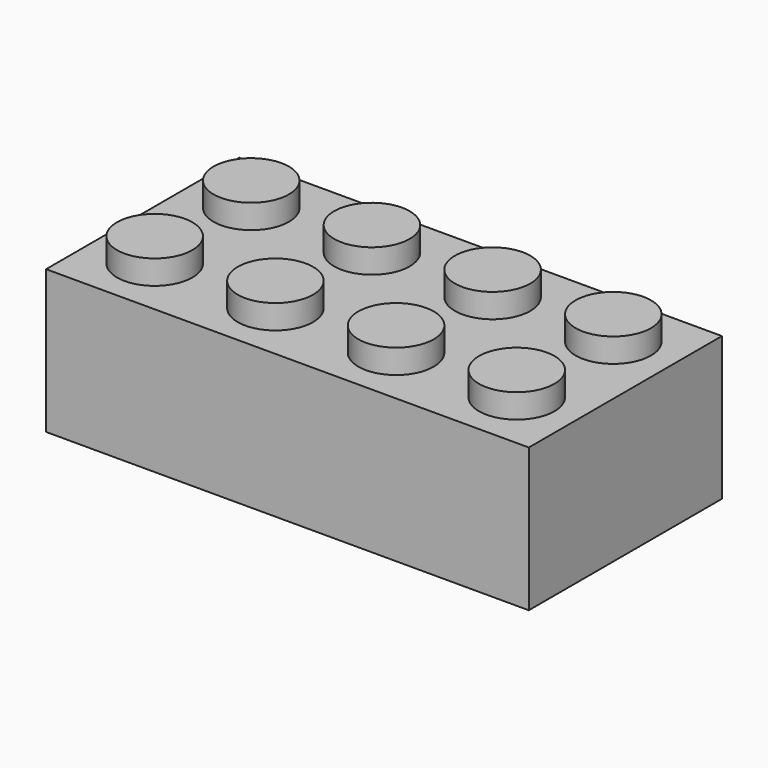
from build123d import *

# Parameters (mm, degrees)
F0_W          = 32
F0_H          = 16
F1_DEPTH      = 9.5
F2_R          = 2.5
F3_DEPTH      = 1.6
F5_T          = -1.5
F4_R          = 3.1568542495
F6_DEPTH      = 9.5
F7_T          = 1
F7_T3_DEPTH   = 10
F7_T5_DEPTH   = 15
F7_T7_DEPTH   = 31
F8_W          = 0.5
F8_H          = 4.8829936233
F9_DEPTH      = 9.5
F10_TEXT_SIZE = 4.2820941114
F11_DEPTH     = 0.7


# Not quite as in the source:
# - a shell that OpenCascade refuses in one call is made with other operations: the cavity is built on its own and cut out
# - Text() gives the source's letters only with a copy of the font that has no kerning and outlines rounded to 1/6400 em; it was checked with that copy


with BuildPart() as f1:
    # F0 (on Top) → F1 (new body)
    with BuildSketch(Plane.XY):
        Rectangle(F0_W, F0_H)
    extrude(amount=F1_DEPTH)

    # F2 (on face) → F3 (join)
    with BuildSketch(Plane.XY.offset(9.5)):
        with Locations((-12, 4)):
            Circle(F2_R)
        with Locations((-12, -4)):
            Circle(F2_R)
        with Locations((-4, 4)):
            Circle(F2_R)
        with Locations((-4, -4)):
            Circle(F2_R)
        with Locations((4, 4)):
            Circle(F2_R)
        with Locations((12, 4)):
            Circle(F2_R)
        with Locations((12, -4)):
            Circle(F2_R)
        with Locations((4, -4)):
            Circle(F2_R)
    extrude(amount=F3_DEPTH)

    # F5
    f5_openings = [f1.faces().sort_by_distance(p)[0] for p in [
        (0, 0, 0),
    ]]
    offset(amount=F5_T, openings=f5_openings, kind=Kind.INTERSECTION)

    # F4 (on face) → F6 (join)
    with BuildSketch(Plane.XY.offset(9.5)):
        Circle(F4_R)
        with Locations((-8, 0)):
            Circle(F4_R)
        with Locations((8, 0)):
            Circle(F4_R)
    extrude(amount=-F6_DEPTH)

    # F7: shell of thickness 1, made by hand


with BuildPart() as f7_core1:
    # F7_t2: copy of F1
    add(f1.part)

    # the walls: a layer under each face that stays
    f7_faces = [f7_core1.faces().sort_by_distance(p)[0] for p in [
        (0, 8, 4.75),
        (0, 0, 9.5),
        (9.5, 4, 10.3),
        (12, 4, 11.1),
        (-6.5, 4, 10.3),
        (-4, 4, 11.1),
        (1.5, 4, 10.3),
        (4, 4, 11.1),
        (1.5, -4, 10.3),
        (4, -4, 11.1),
        (-6.5, -4, 10.3),
        (-4, -4, 11.1),
        (-14.5, 4, 10.3),
        (-12, 4, 11.1),
        (9.5, -4, 10.3),
        (12, -4, 11.1),
        (-14.5, -4, 10.3),
        (-12, -4, 11.1),
        (0, -8, 4.75),
        (-13.7142857143, -6.8571428571, 0),
        (-14.5, 0, 4),
        (-9.6666666667, -4.3333333333, 8),
        (11, 4, 8.8),
        (12, 4, 9.6),
        (3, 4, 8.8),
        (4, 4, 9.6),
        (4.8431457505, 0, 4),
        (-3.1568542495, 0, 4),
        (-5, 4, 8.8),
        (-4, 4, 9.6),
        (-13, 4, 8.8),
        (-12, 4, 9.6),
        (-11.1568542495, 0, 4),
        (11, -4, 8.8),
        (12, -4, 9.6),
        (3, -4, 8.8),
        (4, -4, 9.6),
        (-5, -4, 8.8),
        (-4, -4, 9.6),
        (-13, -4, 8.8),
        (-12, -4, 9.6),
        (0, -6.5, 4),
        (14.5, 0, 4),
        (0, 6.5, 4),
        (-16, 0, 4.75),
        (16, 0, 4.75),
    ]]
    thicken(f7_faces, amount=-F7_T, mode=Mode.SUBTRACT)

    # F7_s4 → F7_t3 (cut)
    with BuildSketch(Plane.XY.offset(-1)):
        Polygon((-14.49, -6.49), (-15.5, -6.5), (-15.5, -7.5), (-14.5, -7.5), align=None)
        Polygon((-14.49, 6.49), (-15.5, 6.5), (-15.5, 7.5), (-14.5, 7.5), align=None)
        Polygon((14.49, -6.49), (14.5, -7.5), (15.5, -7.5), (15.5, -6.5), align=None)
        Polygon((14.49, 6.49), (15.5, 6.5), (15.5, 7.5), (14.5, 7.5), align=None)
    extrude(amount=F7_T3_DEPTH, mode=Mode.SUBTRACT)

    # F7_s6 → F7_t5 (cut)
    with BuildSketch(Plane.XZ.offset(-7.5)):
        Polygon((-14.49, 7.99), (-15.5, 8), (-15.5, 9), (-14.5, 9), align=None)
        Polygon((14.49, 7.99), (14.5, 9), (15.5, 9), (15.5, 8), align=None)
    extrude(amount=F7_T5_DEPTH, mode=Mode.SUBTRACT)

    # F7_s8 → F7_t7 (cut)
    with BuildSketch(Plane.YZ.offset(-15.5)):
        Polygon((-6.49, 7.99), (-6.5, 9), (-7.5, 9), (-7.5, 8), align=None)
        Polygon((6.49, 7.99), (6.5, 9), (7.5, 9), (7.5, 8), align=None)
    extrude(amount=F7_T7_DEPTH, mode=Mode.SUBTRACT)

    # F7_s9 → F7_t10 (revolve, cut)
    with BuildSketch(Plane.XZ.offset(4)):
        Polygon((-9.49, 9.51), (-9.5, 8.5), (-10.5, 8.5), (-10.5, 9.5), align=None)
    revolve(axis=Axis((-12, -4, 9.5), (0, 0, -1)), mode=Mode.SUBTRACT)

    # F7_s11 → F7_t12 (revolve, cut)
    with BuildSketch(Plane.XZ.offset(4)):
        Polygon((14.51, 9.51), (14.5, 8.5), (13.5, 8.5), (13.5, 9.5), align=None)
    revolve(axis=Axis((12, -4, 9.5), (0, 0, -1)), mode=Mode.SUBTRACT)

    # F7_s13 → F7_t14 (revolve, cut)
    with BuildSketch(Plane.XZ.offset(-4)):
        Polygon((-9.49, 9.51), (-9.5, 8.5), (-10.5, 8.5), (-10.5, 9.5), align=None)
    revolve(axis=Axis((-12, 4, 9.5), (0, 0, -1)), mode=Mode.SUBTRACT)

    # F7_s15 → F7_t16 (revolve, cut)
    with BuildSketch(Plane.XZ.offset(4)):
        Polygon((-1.49, 9.51), (-1.5, 8.5), (-2.5, 8.5), (-2.5, 9.5), align=None)
    revolve(axis=Axis((-4, -4, 9.5), (0, 0, -1)), mode=Mode.SUBTRACT)

    # F7_s17 → F7_t18 (revolve, cut)
    with BuildSketch(Plane.XZ.offset(4)):
        Polygon((6.51, 9.51), (6.5, 8.5), (5.5, 8.5), (5.5, 9.5), align=None)
    revolve(axis=Axis((4, -4, 9.5), (0, 0, -1)), mode=Mode.SUBTRACT)

    # F7_s19 → F7_t20 (revolve, cut)
    with BuildSketch(Plane.XZ.offset(-4)):
        Polygon((6.51, 9.51), (6.5, 8.5), (5.5, 8.5), (5.5, 9.5), align=None)
    revolve(axis=Axis((4, 4, 9.5), (0, 0, -1)), mode=Mode.SUBTRACT)

    # F7_s21 → F7_t22 (revolve, cut)
    with BuildSketch(Plane.XZ.offset(-4)):
        Polygon((-1.49, 9.51), (-1.5, 8.5), (-2.5, 8.5), (-2.5, 9.5), align=None)
    revolve(axis=Axis((-4, 4, 9.5), (0, 0, -1)), mode=Mode.SUBTRACT)

    # F7_s23 → F7_t24 (revolve, cut)
    with BuildSketch(Plane.XZ.offset(-4)):
        Polygon((14.51, 9.51), (14.5, 8.5), (13.5, 8.5), (13.5, 9.5), align=None)
    revolve(axis=Axis((12, 4, 9.5), (0, 0, -1)), mode=Mode.SUBTRACT)

    # F7_s25 → F7_t26 (revolve, cut)
    with BuildSketch(Plane.XZ):
        Polygon((-4.8331457505, 7.99), (-4.8431457505, 9), (-5.8431457505, 9), (-5.8431457505, 8), align=None)
    revolve(axis=Axis((-8, 0, 8), (0, 0, 1)), mode=Mode.SUBTRACT)

    # F7_s27 → F7_t28 (revolve, cut)
    with BuildSketch(Plane.XZ):
        Polygon((3.1668542495, 7.99), (3.1568542495, 9), (2.1568542495, 9), (2.1568542495, 8), align=None)
    revolve(axis=Axis((0, 0, 8), (0, 0, 1)), mode=Mode.SUBTRACT)

    # F7_s29 → F7_t30 (revolve, cut)
    with BuildSketch(Plane.XZ):
        Polygon((11.1668542495, 7.99), (11.1568542495, 9), (10.1568542495, 9), (10.1568542495, 8), align=None)
    revolve(axis=Axis((8, 0, 8), (0, 0, 1)), mode=Mode.SUBTRACT)

    # F7_s31 → F7_t32 (revolve, cut)
    with BuildSketch(Plane.XZ.offset(-4)):
        Polygon((12.99, 9.59), (14, 9.6), (14, 10.6), (13, 10.6), align=None)
    revolve(axis=Axis((12, 4, 9.6), (0, 0, -1)), mode=Mode.SUBTRACT)

    # F7_s33 → F7_t34 (revolve, cut)
    with BuildSketch(Plane.XZ.offset(-4)):
        Polygon((4.99, 9.59), (6, 9.6), (6, 10.6), (5, 10.6), align=None)
    revolve(axis=Axis((4, 4, 9.6), (0, 0, -1)), mode=Mode.SUBTRACT)

    # F7_s35 → F7_t36 (revolve, cut)
    with BuildSketch(Plane.XZ.offset(-4)):
        Polygon((-3.01, 9.59), (-2, 9.6), (-2, 10.6), (-3, 10.6), align=None)
    revolve(axis=Axis((-4, 4, 9.6), (0, 0, -1)), mode=Mode.SUBTRACT)

    # F7_s37 → F7_t38 (revolve, cut)
    with BuildSketch(Plane.XZ.offset(-4)):
        Polygon((-11.01, 9.59), (-10, 9.6), (-10, 10.6), (-11, 10.6), align=None)
    revolve(axis=Axis((-12, 4, 9.6), (0, 0, -1)), mode=Mode.SUBTRACT)

    # F7_s39 → F7_t40 (revolve, cut)
    with BuildSketch(Plane.XZ.offset(4)):
        Polygon((12.99, 9.59), (14, 9.6), (14, 10.6), (13, 10.6), align=None)
    revolve(axis=Axis((12, -4, 9.6), (0, 0, -1)), mode=Mode.SUBTRACT)

    # F7_s41 → F7_t42 (revolve, cut)
    with BuildSketch(Plane.XZ.offset(4)):
        Polygon((4.99, 9.59), (6, 9.6), (6, 10.6), (5, 10.6), align=None)
    revolve(axis=Axis((4, -4, 9.6), (0, 0, -1)), mode=Mode.SUBTRACT)

    # F7_s43 → F7_t44 (revolve, cut)
    with BuildSketch(Plane.XZ.offset(4)):
        Polygon((-3.01, 9.59), (-2, 9.6), (-2, 10.6), (-3, 10.6), align=None)
    revolve(axis=Axis((-4, -4, 9.6), (0, 0, -1)), mode=Mode.SUBTRACT)

    # F7_s45 → F7_t46 (revolve, cut)
    with BuildSketch(Plane.XZ.offset(4)):
        Polygon((-11.01, 9.59), (-10, 9.6), (-10, 10.6), (-11, 10.6), align=None)
    revolve(axis=Axis((-12, -4, 9.6), (0, 0, -1)), mode=Mode.SUBTRACT)


with BuildPart() as f1_1:
    add(f1.part)

    # what is left inside the walls is the cavity
    f7_cavity = [f7_core1.part.solids().sort_by_distance(p)[0] for p in [
        (-10.146854, 0, 5.666667),
        (-2.146854, 0, 5.666667),
        (5.853146, 0, 5.666667),
    ]]
    add(f7_cavity, mode=Mode.SUBTRACT)

    # F8 (on face) → F9 (join)
    with BuildSketch(Plane.XY.offset(9.5)):
        with Locations((0.25, 5.5585031884)):
            Rectangle(F8_W, F8_H)
        with Locations((-0.25, 5.5585031884)):
            Rectangle(F8_W, F8_H)
        with Locations((0.25, -5.5585031884)):
            Rectangle(F8_W, F8_H)
        with Locations((-0.25, -5.5585031884)):
            Rectangle(F8_W, F8_H)
    extrude(amount=-F9_DEPTH)

    # F10 (on face) → F11 (join)
    with BuildSketch(Plane(origin=(0, 8, 0), x_dir=(-1, 0, 0), z_dir=(0, 1, 0))):
        with Locations((-9.7880344838, 3.3240302)):
            Text('HUBBALL', F10_TEXT_SIZE, font='Open Sans', font_style=FontStyle.BOLD, text_align=(TextAlign.LEFT, TextAlign.BOTTOM))
    extrude(amount=F11_DEPTH)


solid = f1_1.part
